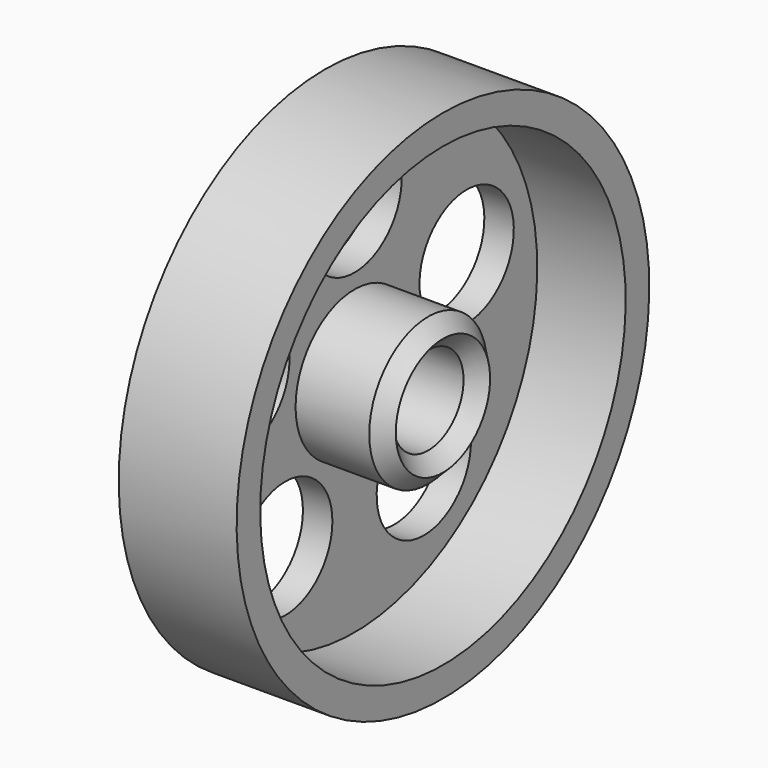
from build123d import *

# Parameters (mm, degrees)
F0_W            = 8
F0_H            = 17.5
F3_D            = 6
F4_T            = -2
F6_D            = 8
F6_COPIES_COUNT = 5
F7_SIZE         = 0.99999


# Not quite as in the source:
# - a fillet or chamfer is up to 0.001 mm smaller than in the source, because OpenCascade refuses the exact size
# - a pattern or mirror of a feature is missing from the dataset's text; its kind, count and spacing are read off the source's solid


with BuildPart() as f1:
    # F0 (on Front) → F1 (revolve)
    with BuildSketch(Plane.XZ):
        with Locations((4, 8.75)):
            Rectangle(F0_W, F0_H)
    revolve(axis=Axis((4, 0, 0), (1, 0, 0)))

    # F3 (through all)
    with Locations(Plane(origin=(0, 0, 0), x_dir=(0, 1, 0), z_dir=(-1, 0, 0))):
        with Locations((0, 0)):
            Hole(F3_D / 2)

    # F4
    f4_openings = [f1.faces().sort_by_distance(p)[0] for p in [
        (8, 0, -17.005025),
    ]]
    offset(amount=F4_T, openings=f4_openings)

    # F6 (through all)
    with Locations(Plane(origin=(0, 0, 0), x_dir=(0, 1, 0), z_dir=(-1, 0, 0))):
        with Locations((0, -10)):
            f6 = Hole(F6_D / 2)

    # F6_copies: F6 ×5 about axis
    f6_copies_axis = Axis((0, 0, 0), (1, 0, 0))
    for i in range(1, F6_COPIES_COUNT):
        add(f6.rotate(f6_copies_axis, i * 360 / F6_COPIES_COUNT), mode=Mode.SUBTRACT)

    # F7 (size 1 in the source; OpenCascade refuses exactly that, so slightly less here)
    f7_edges = [f1.edges().sort_by_distance(p)[0] for p in [
        (8, -3, 0),
        (8, -5, 0),
    ]]
    chamfer(f7_edges, length=F7_SIZE)


solid = f1.part
